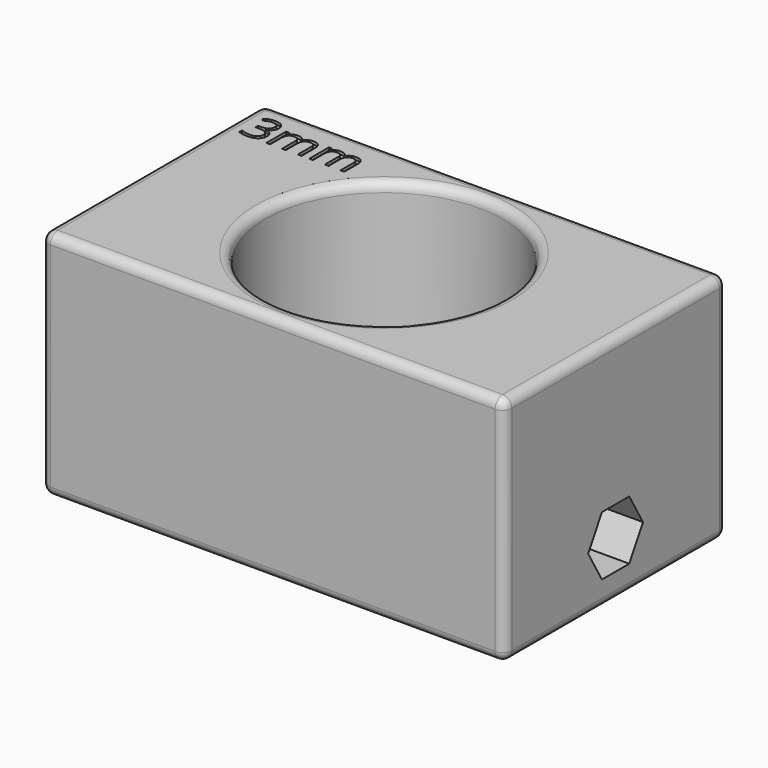
from build123d import *

# Parameters (mm, degrees)
F0_R          = 12.85
F1_DEPTH      = 3
F0_W          = 50
F0_H          = 30
F2_DEPTH      = 25
F3_R          = 1
F5_START      = -15
F5_DEPTH      = 25
F6_START      = 15
F6_DEPTH      = 25
F7_R          = 1.5
F8_DEPTH      = 50
F8_DEPTH_BACK = 50
F10_START     = 24.7
F9_TEXT_SIZE  = 4.9673371709
F10_DEPTH     = 5.3


# Not quite as in the source:
# - Text() gives the source's letters only with a copy of the font that has no kerning and outlines rounded to 1/6400 em; it was checked with that copy


with BuildPart() as f1:
    # F0 (on Top) → F1 (new body)
    with BuildSketch(Plane.XY):
        Circle(F0_R)
    extrude(amount=F1_DEPTH)

    # F0 (on Top) → F2 (join)
    with BuildSketch(Plane.XY):
        Rectangle(F0_W, F0_H)
        Circle(F0_R, mode=Mode.SUBTRACT)
    extrude(amount=F2_DEPTH)

    # F3
    f3_edges = [f1.edges().sort_by_distance(p)[0] for p in [
        (-25, 15, 12.5),
        (25, 15, 12.5),
        (-25, -15, 12.5),
        (25, -15, 12.5),
        (25, 0, 0),
        (0, 15, 0),
        (-25, 0, 0),
        (0, -15, 0),
        (0, -15, 25),
        (0, 15, 25),
        (-25, 0, 25),
        (25, 0, 25),
        (-12.85, 0, 25),
    ]]
    fillet(f3_edges, radius=F3_R)

    # F4 (on Right) → F5 (cut)
    with BuildSketch(Plane.YZ.offset(F5_START)):
        Polygon((0, 2.8), (1.8475208614, 2.8), (3.6950417228, 6), (1.8475208614, 9.2), (-1.8475208614, 9.2), (-3.6950417228, 6), (-1.8475208614, 2.8), align=None)
    extrude(amount=-F5_DEPTH, mode=Mode.SUBTRACT)

    # F4 (on Right) → F6 (cut)
    with BuildSketch(Plane.YZ.offset(F6_START)):
        Polygon((0, 2.8), (1.8475208614, 2.8), (3.6950417228, 6), (1.8475208614, 9.2), (-1.8475208614, 9.2), (-3.6950417228, 6), (-1.8475208614, 2.8), align=None)
    extrude(amount=F6_DEPTH, mode=Mode.SUBTRACT)

    # F7 (on Right) → F8 (cut, two sides)
    with BuildSketch(Plane.YZ) as f8_sk:
        with Locations((0, 6)):
            Circle(F7_R)
    extrude(amount=-F8_DEPTH, mode=Mode.SUBTRACT)
    extrude(f8_sk.sketch, amount=F8_DEPTH_BACK, mode=Mode.SUBTRACT)

    # F9 (on Top) → F10 (cut)
    with BuildSketch(Plane.XY.offset(F10_START)):
        with Locations((-23.5, 9.4235172369)):
            Text('3mm', F9_TEXT_SIZE, font='Open Sans', text_align=(TextAlign.LEFT, TextAlign.BOTTOM))
    extrude(amount=F10_DEPTH, mode=Mode.SUBTRACT)


solid = f1.part
